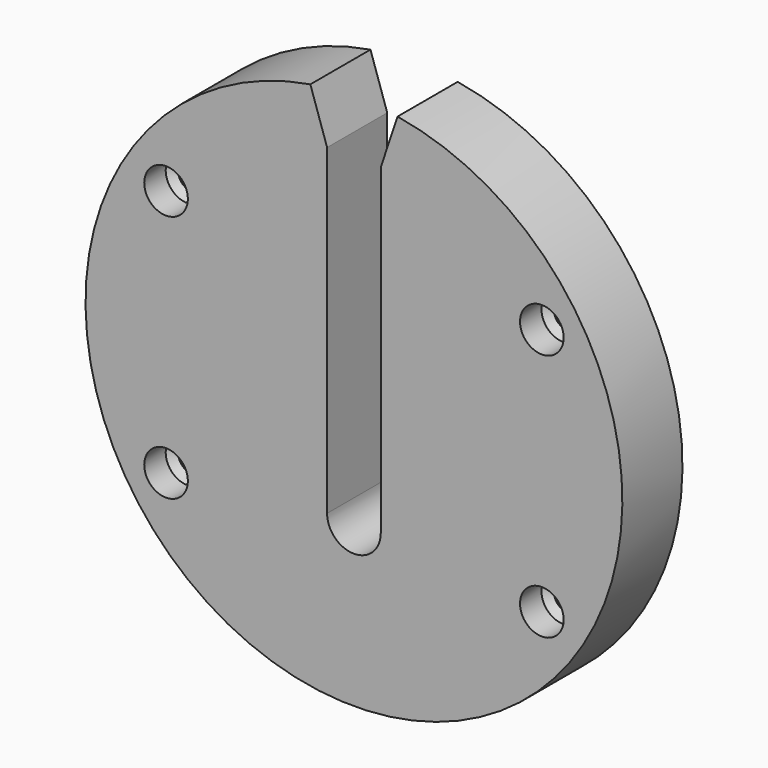
from build123d import *

# Parameters (mm, degrees)
F0_R           = 63.5
F1_DEPTH       = 17.78
F2_D           = 6.35
F2_CBORE_D     = 15.875
F2_CBORE_DEPTH = 3.175
F4_D           = 10.31875
F4_DEPTH       = 6.35
F4_TIP         = 3.1000652563
F6_DEPTH       = 25.4


# Not quite as in the source:
# - a length typed as a fraction of an inch, garbled in the dataset ("3 / 203.2 mm" for 3/8 in), is restored
# - a feature names something its author has since deleted; it is built from what else it names


with BuildPart() as f1:
    # F0 (on Front) → F1 (new body)
    with BuildSketch(Plane.XZ):
        Circle(F0_R)
    extrude(amount=F1_DEPTH)

    # F2 (through all)
    with Locations(Plane(origin=(0, 0, 0), x_dir=(1, 0, 0), z_dir=(0, 1, 0))):
        with Locations((44.45, -29.36875), (-44.45, -29.36875), (-44.45, 29.36875), (44.45, 29.36875)):
            CounterBoreHole(F2_D / 2, F2_CBORE_D / 2, F2_CBORE_DEPTH)

    # F4
    with Locations(Plane.XZ.offset(17.78)):
        with Locations((-44.45, 29.36875), (44.45, 29.36875), (44.45, -29.36875), (-44.45, -29.36875)):
            Hole(F4_D / 2, depth=F4_DEPTH)
            with Locations((0, 0, -(F4_DEPTH + F4_TIP / 2))):  # 118° drill point
                Cone(0, F4_D / 2, F4_TIP, mode=Mode.SUBTRACT)

    # F5 (on face) → F6 (cut)
    with BuildSketch(Plane.XZ.offset(17.78)):
        with BuildLine():
            Line((-10.3124, 62.6570379625), (-6.35, 50.8))
            Line((-6.35, 50.8), (-6.35, -25.4))
            ThreePointArc((-6.35, -25.4), (0, -31.75), (6.35, -25.4))
            Line((6.35, -25.4), (6.35, 50.8))
            Line((6.35, 50.8), (10.3124, 62.6570379625))
            ThreePointArc((10.3124, 62.6570379625), (0, 63.5), (-10.3124, 62.6570379625))
        make_face()
    extrude(amount=-F6_DEPTH, mode=Mode.SUBTRACT)


solid = f1.part
